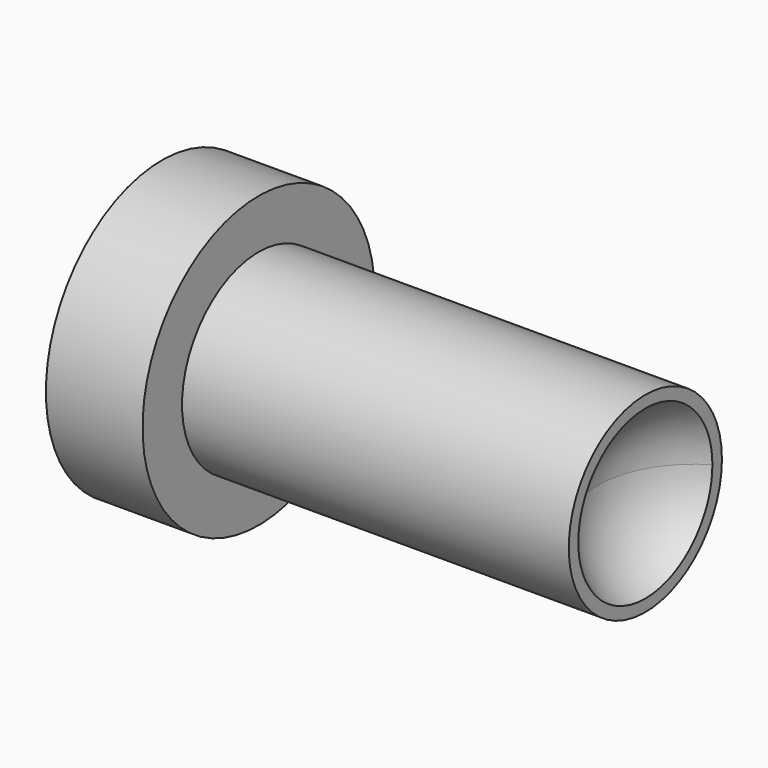
from build123d import *
from build123d import SkipClean  # not in build123d's __all__

# Parameters (mm, degrees)
F0_R      = 0.495
F1_DEPTH  = 2
F0_R_2    = 0.75
F1_FACE_R = 0.495
F2_DEPTH  = 0.5


with BuildPart() as f1:
    # F0 (on Right) → F1 (new body)
    with BuildSketch(Plane.YZ):
        Circle(F0_R)
    extrude(amount=F1_DEPTH)

    # F0 (on Right) + F1_face (on face) → F2 (join)
    with BuildSketch(Plane.YZ):
        Circle(F0_R_2)
        Circle(F0_R, mode=Mode.SUBTRACT)
    with BuildSketch(Plane(origin=(0, 0, 0), x_dir=(0, 1, 0), z_dir=(-1, 0, 0))):
        Circle(F1_FACE_R)
    extrude(amount=-F2_DEPTH, dir=(1, 0, 0))

    # F3 (on Top) → F4 (revolve, cut)
    with BuildSketch(Plane.XY):
        with BuildLine():
            Line((2.25, -0.5), (2.25, 0.5))
            ThreePointArc((2.25, 0.5), (1.75, 0), (2.25, -0.5))
        make_face()
    with SkipClean():  # cleaning this boolean's faces spoils the solid; the shape is the same uncleaned
        revolve(axis=Axis((2.25, 0.0427489867, 0), (0, -1, 0)), mode=Mode.SUBTRACT)


solid = f1.part
